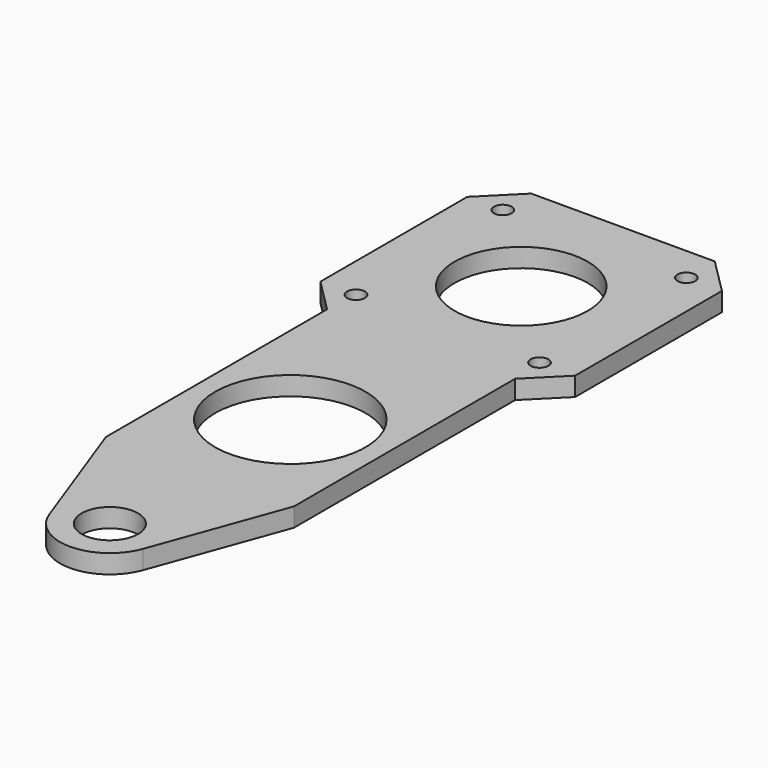
from build123d import *

# Parameters (mm, degrees)
F0_R         = 4.7625
F0_R_2       = 1.5
F0_R_3       = 11.2530001
F1_DEPTH     = 3.175
F2_T1_DEPTH  = 34.0506804732
F2_T6_DEPTH  = 34.0506804732
F2_T11_DEPTH = 34.0506804732


# Not quite as in the source:
# - a fillet or chamfer that OpenCascade refuses, or shapes differently, is made with other operations: its cross-section is extruded or revolved along the edge and cut away or added


with BuildPart() as f1:
    # F0 (on Top) → F1 (new body)
    with BuildSketch(Plane.XY):
        with BuildLine():
            Line((15.875, 0), (12.7, 0))
            ThreePointArc((12.7, 0), (0, -12.7), (-12.7, 0))
            Line((-12.7, 0), (-15.875, 0))
            Line((-15.875, 0), (-15.875, -19.0989050379))
            Line((-15.875, -19.0989050379), (-7.9111435612, -40.9794207753))
            ThreePointArc((-7.9111435612, -40.9794207753), (0, -46.5188631327), (7.9111435612, -40.9794207753))
            Line((7.9111435612, -40.9794207753), (15.875, -19.0989050379))
            Line((15.875, -19.0989050379), (15.875, 0))
        make_face()
        with Locations((0, -38.1)):
            Circle(F0_R, mode=Mode.SUBTRACT)
        with BuildLine():
            ThreePointArc((-12.7, 0), (0, 12.7), (12.7, 0))
            Line((12.7, 0), (15.875, 0))
            Line((15.875, 0), (15.875, 27.2180678568))
            Line((15.875, 27.2180678568), (21.5029923, 27.2180678568))
            Line((21.5029923, 27.2180678568), (21.5029923, 70.2240524568))
            Line((21.5029923, 70.2240524568), (-21.5029923, 70.2240524568))
            Line((-21.5029923, 70.2240524568), (-21.5029923, 27.2180678568))
            Line((-21.5029923, 27.2180678568), (-15.875, 27.2180678568))
            Line((-15.875, 27.2180678568), (-15.875, 0))
            Line((-15.875, 0), (-12.7, 0))
        make_face()
        with Locations((-15.4999944, 33.2210657568)):
            Circle(F0_R_2, mode=Mode.SUBTRACT)
        with Locations((-15.4999944, 64.2210545568)):
            Circle(F0_R_2, mode=Mode.SUBTRACT)
        with Locations((15.4999944, 33.2210657568)):
            Circle(F0_R_2, mode=Mode.SUBTRACT)
        with Locations((0, 48.7210601568)):
            Circle(F0_R_3, mode=Mode.SUBTRACT)
        with Locations((15.4999944, 64.2210545568)):
            Circle(F0_R_2, mode=Mode.SUBTRACT)
    extrude(amount=F1_DEPTH)

    # F2: chamfer of 6.0030106 on 4 edges, made by hand

    # F2_s2 → F2_t1 (cut)
    with BuildSketch(Plane.XY.offset(-15.4378402366)):
        Polygon((21.5029923, 64.2210418568), (15.4999817, 70.2240524568), (21.5029923, 70.2240524568), align=None)
        Polygon((-15.4999817, 70.2240524568), (-21.5029923, 64.2210418568), (-21.5029923, 70.2240524568), align=None)
    extrude(amount=F2_T1_DEPTH, mode=Mode.SUBTRACT)


with BuildPart() as f2_tool4:
    # F2_s5 → F2_t6 (new body)
    with BuildSketch(Plane.XY.offset(-15.4378402366)):
        Polygon((15.4999817, 27.2180678568), (21.5029923, 33.2210784568), (21.5029923, 27.2180678568), align=None)
    extrude(amount=F2_T6_DEPTH)

    split(bisect_by=Plane.YZ.offset(15.875), keep=Keep.TOP)


with BuildPart() as f1_1:
    add(f1.part)

    # F2_t3: cut F2_tool4
    add(f2_tool4.part, mode=Mode.SUBTRACT)


with BuildPart() as f2_tool9:
    # F2_s10 → F2_t11 (new body)
    with BuildSketch(Plane.XY.offset(-15.4378402366)):
        Polygon((-21.5029923, 33.2210784568), (-15.4999817, 27.2180678568), (-21.5029923, 27.2180678568), align=None)
    extrude(amount=F2_T11_DEPTH)

    split(bisect_by=Plane.YZ.offset(-15.875), keep=Keep.BOTTOM)


with BuildPart() as f1_2:
    add(f1_1.part)

    # F2_t8: cut F2_tool9
    add(f2_tool9.part, mode=Mode.SUBTRACT)


solid = f1_2.part
